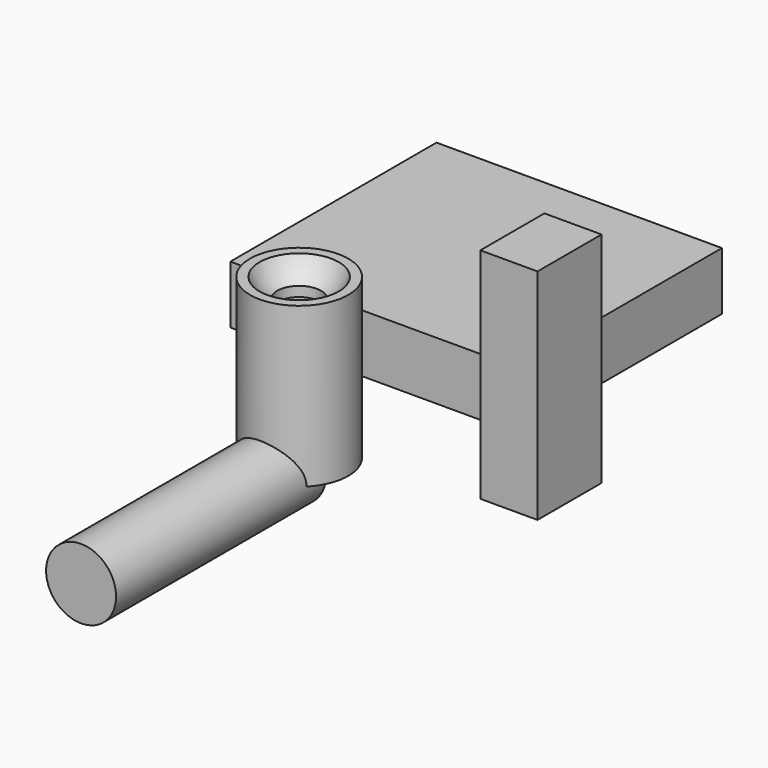
from build123d import *

# Parameters (mm, degrees)
F2_W      = 4
F2_H      = 30
F7_R      = 2.5
F8_DEPTH  = 25
F9_W      = 6.5303985029
F9_H      = 9.1462465934
F10_DEPTH = 25
F11_ANGLE = 90
F13_W     = 32.6160658151
F13_H     = 29.4494852424
F14_DEPTH = 6.6303107317


# Not quite as in the source:
# - a feature names something its author has since deleted; it is built from what else it names
# - the program builds the solid bodies; features that only make, move or delete a surface that nothing else refers to are left out


with BuildPart() as f3:
    # F2 (on Top) → F3 (revolve)
    with BuildSketch(Plane.XY):
        with Locations((-2, -15.5)):
            Rectangle(F2_W, F2_H)
    revolve(axis=Axis((0, -15.5, 0), (0, 1, 0)))


with BuildPart() as f5:
    # F4 (on Top) → F5 (revolve)
    with BuildSketch(Plane.XY):
        with BuildLine():
            ThreePointArc((0, 0), (-2.6864980417, 0.7830427709), (-4.5315389352, 2.8869086913))
            Line((-4.5315389352, 2.8869086913), (-5.6155894723, 2.8869086913))
            Line((-5.6155894723, 2.8869086913), (-5.6155894723, -15.3195205119))
            Line((-5.6155894723, -15.3195205119), (-4.2155894723, -15.3195205119))
            Line((-4.2155894723, -15.3195205119), (-4.2155894723, -0.3195205119))
            Line((-4.2155894723, -0.3195205119), (-2.7753741232, -0.3195205119))
            ThreePointArc((-2.7753741232, -0.3195205119), (-1.4287891602, -0.8273974925), (0, -1))
            Line((0, -1), (0, 0))
        make_face()
    revolve(axis=Axis((0, -0.5, 0), (0, -1, 0)))

    # F7 (on offset) → F8 (cut)
    with BuildSketch(Plane.XZ.offset(1)):
        Circle(F7_R)
    extrude(amount=-F8_DEPTH, mode=Mode.SUBTRACT)


with BuildPart() as f10:
    # F9 (on Top) → F10 (new body)
    with BuildSketch(Plane.XY):
        with Locations((20.8507301286, 9.1232920531)):
            Rectangle(F9_W, F9_H)
    extrude(amount=F10_DEPTH)


with BuildPart() as f5_1:
    # F11: moved
    add(f5.part.rotate(Axis((20.8507301286, 4.5501687564, 25), (1, 0, 0)), F11_ANGLE))


with BuildPart() as f5_2:
    # F12: moved
    add(f5_1.part.moved(Location((0, 0, 1.5))))


with BuildPart() as f14:
    # F13 (on Top) → F14 (new body, through all)
    with BuildSketch(Plane.XY):
        with Locations((-4.2099980637, 31.1885289848)):
            Rectangle(F13_W, F13_H)
    extrude(amount=F14_DEPTH)


with BuildPart() as f5_3:
    # F15: moved
    add(f5_2.part.moved(Location((0, 0, -6.6303107317))))


with BuildPart() as f5_4:
    # F16: moved
    add(f5_3.part.moved(Location((0, -28.9, 0))))


solid = Compound([f3.part, f10.part, f14.part, f5_4.part])
